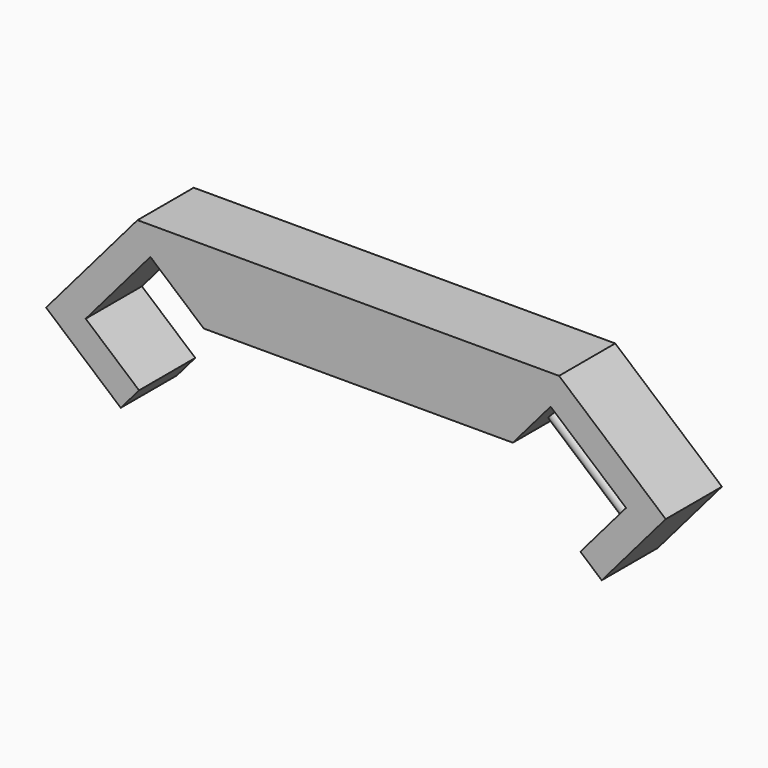
from build123d import *

# Parameters (mm, degrees)
F1_DEPTH = 63.5
F2_R     = 5.6131699843
F3_DEPTH = 107.696


# Not quite as in the source:
# - the program builds the solid bodies; features that only make, move or delete a surface that nothing else refers to are left out


with BuildPart() as f1:
    # F0 (on Front) → F1 (new body)
    with BuildSketch(Plane.XZ):
        Polygon((46.8248670694, 121.5258430131), (-35.8149119383, 25.0910623293), (31.6894345404, -32.7567829762), (48.2173903419, -13.4698268394), (0, 27.8500626645), (58.4593796701, 96.0680265203), (106.676770012, 54.7481370164), (386.0897425486, 54.7481370164), (420.2281583997, 94.5852552302), (488.444735815, 36.1270636701), (447.1248463111, -12.0903266718), (466.4118024479, -28.6182824733), (524.2596477533, 38.8860640054), (427.8248670694, 121.5258430131), align=None)
    extrude(amount=F1_DEPTH)

    # F2 (on face) → F3 (join)
    with BuildSketch(Plane(origin=(195.5607291239, 0, -167.5857540484), x_dir=(0, 1, 0), z_dir=(0.7593289818, 0, -0.6507069213))):
        with Locations((-31.75, 311.8531148615)):
            Circle(F2_R)
    extrude(amount=F3_DEPTH)


solid = f1.part
